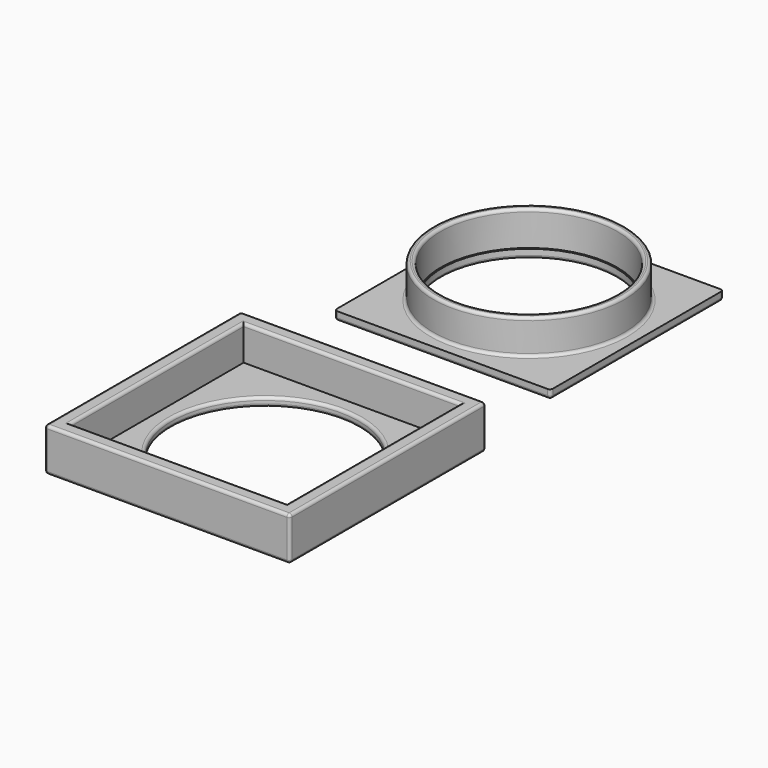
from build123d import *

# Parameters (mm, degrees)
F0_R     = 33.2
F0_R_2   = 30.7
F1_DEPTH = 15
F0_W     = 85.1
F0_H     = 85.1
F0_W_2   = 75.1
F0_H_2   = 75.1
F0_W_3   = 75
F0_H_3   = 75
F0_R_3   = 30.2
F2_DEPTH = 3
F0_R_4   = 32.5
F3_R     = 1
F3_2_R   = 1


# Not quite as in the source:
# - a feature names something its author has since deleted; it is built from what else it names


with BuildPart() as f1:
    # F0 (on Top) → F1 (new body)
    with BuildSketch(Plane.XY):
        with Locations((37.5, 37.5)):
            Circle(F0_R)
        with Locations((37.5, 37.5)):
            Circle(F0_R_2, mode=Mode.SUBTRACT)
    extrude(amount=F1_DEPTH)

    # F0 (on Top) → F2 (join)
    with BuildSketch(Plane.XY):
        with Locations((37.5, 37.5)):
            Rectangle(F0_W_3, F0_H_3)
        with Locations((37.5, 37.5)):
            Circle(F0_R, mode=Mode.SUBTRACT)
        with Locations((37.5, 37.5)):
            Circle(F0_R_2)
        with Locations((37.5, 37.5)):
            Circle(F0_R_3, mode=Mode.SUBTRACT)
    extrude(amount=F2_DEPTH)

    # F3
    f3_edges = [f1.edges().sort_by_distance(p)[0] for p in [
        (6.8, 37.5, 15),
        (4.3, 37.5, 15),
        (37.5, 0, 0),
        (75, 37.5, 0),
        (37.5, 75, 0),
        (0, 37.5, 0),
        (7.3, 37.5, 0),
        (75, 75, 1.5),
        (0, 75, 1.5),
        (0, 0, 1.5),
        (75, 0, 1.5),
        (4.3, 37.5, 3),
    ]]
    fillet(f3_edges, radius=F3_R)


with BuildPart() as f1b:
    # F0 (on Top) → F1, piece 2 (new body)
    with BuildSketch(Plane.XY):
        with Locations((37.55, -76.9540923819)):
            Rectangle(F0_W, F0_H)
        with Locations((37.55, -76.9540924937)):
            Rectangle(F0_W_2, F0_H_2, mode=Mode.SUBTRACT)
    extrude(amount=F1_DEPTH)

    # F0 (on Top) → F2, piece 2 (join)
    with BuildSketch(Plane.XY):
        with Locations((37.55, -76.9540924937)):
            Rectangle(F0_W_2, F0_H_2)
        with Locations((37.55, -76.9540923819)):
            Circle(F0_R_4, mode=Mode.SUBTRACT)
    extrude(amount=F2_DEPTH)

    # F3#2
    f3_2_edges = [f1b.edges().sort_by_distance(p)[0] for p in [
        (80.1, -76.954092, 15),
        (37.55, -34.404092, 15),
        (-5, -76.954092, 15),
        (37.55, -119.504092, 15),
        (-5, -119.504092, 7.5),
        (80.1, -119.504092, 7.5),
        (80.1, -34.404092, 7.5),
        (-5, -34.404092, 7.5),
        (37.55, -34.404092, 0),
        (80.1, -76.954092, 0),
        (5.05, -76.954092, 0),
        (-5, -76.954092, 0),
        (37.55, -119.504092, 0),
        (5.05, -76.954092, 3),
        (0, -76.954092, 15),
        (37.55, -39.404092, 15),
        (75.1, -76.954092, 15),
        (37.55, -114.504092, 15),
    ]]
    fillet(f3_2_edges, radius=F3_2_R)


solid = Compound([f1.part, f1b.part])
